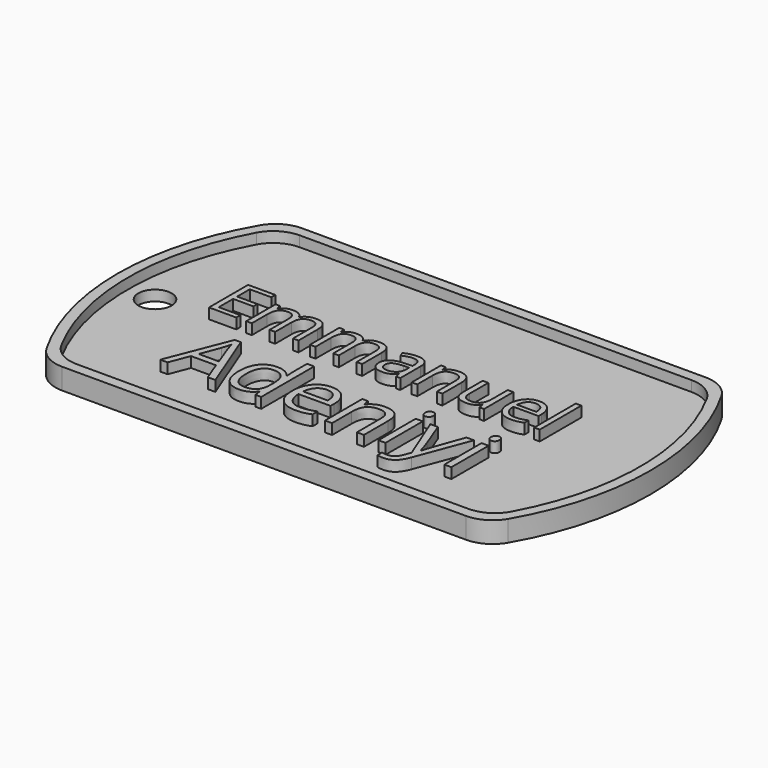
from build123d import *

# Parameters (mm, degrees)
F1_DEPTH     = 1
F3_DEPTH     = 1
F4_R         = 1.5875
F5_DEPTH     = 1
F7_TEXT_SIZE = 8.2946870761
F6_TEXT_SIZE = 6.5250244612
F8_DEPTH     = 1


# Not quite as in the source:
# - Text() gives the source's letters only with a copy of the font that has no kerning and outlines rounded to 1/6400 em; it was checked with that copy


with BuildPart() as f1:
    # F0 (on Top) → F1 (new body)
    with BuildSketch(Plane.XY):
        with BuildLine():
            ThreePointArc((-19.2474145991, 14.2875), (-20.8349145991, 13.862130657), (-21.9970452561, 12.7))
            ThreePointArc((-21.9970452561, 12.7), (-25.4, 0), (-21.9970452561, -12.7))
            ThreePointArc((-21.9970452561, -12.7), (-20.8349145991, -13.862130657), (-19.2474145991, -14.2875))
            Line((-19.2474145991, -14.2875), (19.2474145991, -14.2875))
            ThreePointArc((19.2474145991, -14.2875), (20.8349145991, -13.862130657), (21.9970452561, -12.7))
            ThreePointArc((21.9970452561, -12.7), (25.4, 0), (21.9970452561, 12.7))
            ThreePointArc((21.9970452561, 12.7), (20.8349145991, 13.862130657), (19.2474145991, 14.2875))
            Line((19.2474145991, 14.2875), (-19.2474145991, 14.2875))
        make_face()
    extrude(amount=F1_DEPTH)

    # F2 (on face) → F3 (join)
    with BuildSketch(Plane.XY.offset(1)):
        with BuildLine():
            Line((19.2474145991, 14.2875), (-19.2474145991, 14.2875))
            ThreePointArc((-19.2474145991, 14.2875), (-20.8349145991, 13.862130657), (-21.9970452561, 12.7))
            ThreePointArc((-21.9970452561, 12.7), (-25.4, 0), (-21.9970452561, -12.7))
            ThreePointArc((-21.9970452561, -12.7), (-20.8349145991, -13.862130657), (-19.2474145991, -14.2875))
            Line((-19.2474145991, -14.2875), (19.2474145991, -14.2875))
            ThreePointArc((19.2474145991, -14.2875), (20.8349145991, -13.862130657), (21.9970452561, -12.7))
            ThreePointArc((21.9970452561, -12.7), (25.4, 0), (21.9970452561, 12.7))
            ThreePointArc((21.9970452561, 12.7), (20.8349145991, 13.862130657), (19.2474145991, 14.2875))
        make_face()
        with BuildLine():
            ThreePointArc((-21.4526124879, 11.6252061249), (-20.2856017842, 12.8404540819), (-18.6611352482, 13.2875))
            Line((-18.6611352482, 13.2875), (18.6611352482, 13.2875))
            ThreePointArc((18.6611352482, 13.2875), (20.2856017842, 12.8404540819), (21.4526124879, 11.6252061249))
            ThreePointArc((21.4526124879, 11.6252061249), (24.4, 0), (21.4526124879, -11.6252061249))
            ThreePointArc((21.4526124879, -11.6252061249), (20.2856017842, -12.8404540819), (18.6611352482, -13.2875))
            Line((18.6611352482, -13.2875), (-18.6611352482, -13.2875))
            ThreePointArc((-18.6611352482, -13.2875), (-20.2856017842, -12.8404540819), (-21.4526124879, -11.6252061249))
            ThreePointArc((-21.4526124879, -11.6252061249), (-24.4, 0), (-21.4526124879, 11.6252061249))
        make_face(mode=Mode.SUBTRACT)
    extrude(amount=F3_DEPTH)

    # F4 (on face) → F5 (cut)
    with BuildSketch(Plane.XY.offset(1)):
        with Locations((-21.821282804, 0)):
            Circle(F4_R)
    extrude(amount=-F5_DEPTH, mode=Mode.SUBTRACT)

    # F7 (on face) + F6 (on face) → F8 (join)
    with BuildSketch(Plane.XY.offset(1)):
        with Locations((-14.250991866, -8.8374232873)):
            Text('Adeniyi', F7_TEXT_SIZE, font='Open Sans', text_align=(TextAlign.LEFT, TextAlign.BOTTOM))
    with BuildSketch(Plane.XY.offset(1)):
        with Locations((-17.31595397, 0)):
            Text('Emmanuel', F6_TEXT_SIZE, font='Open Sans', text_align=(TextAlign.LEFT, TextAlign.BOTTOM))
    extrude(amount=F8_DEPTH)


solid = f1.part
